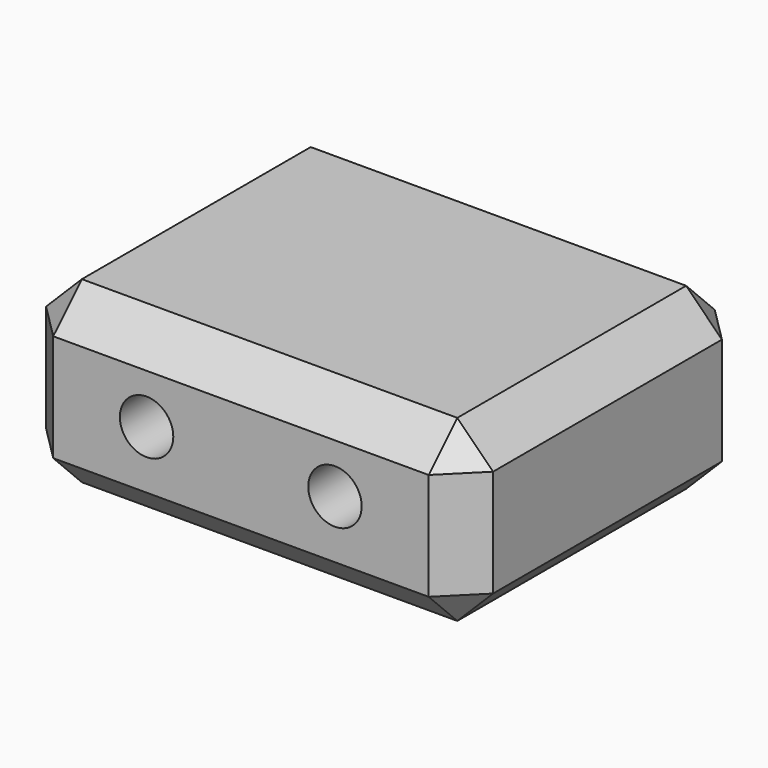
from build123d import *

# Parameters (mm, degrees)
F1_DEPTH = 5
F3_SIZE  = 1
F4_R     = 0.7470588235
F5_DEPTH = 7.5


# Not quite as in the source:
# - a feature names something its author has since deleted; it is built from what else it names


with BuildPart() as f1:
    # F0 (on Top) → F1 (new body)
    with BuildSketch(Plane.XY):
        Polygon((9.4699421152, -1.9223576039), (-3.0300578848, -1.9223576039), (-3.0300578848, -6.9223576039), (-3.0300578848, -11.9223576039), (9.4699421152, -11.9223576039), align=None)
    extrude(amount=F1_DEPTH)

    # F3
    f3_edges = [f1.edges().sort_by_distance(p)[0] for p in [
        (3.219942, -11.922358, 5),
        (9.469942, -6.922358, 5),
        (-3.030058, -1.922358, 2.5),
        (-3.030058, -11.922358, 2.5),
        (9.469942, -11.922358, 2.5),
        (9.469942, -6.922358, 0),
        (3.219942, -11.922358, 0),
        (9.469942, -1.922358, 2.5),
        (-3.030058, -6.922358, 5),
        (3.219942, -1.922358, 5),
        (3.219942, -1.922358, 0),
        (-3.030058, -6.922358, 0),
    ]]
    chamfer(f3_edges, length=F3_SIZE)

    # F4 (on face) → F5 (cut)
    with BuildSketch(Plane.XZ.offset(11.9223576039)):
        with Locations((0.5804465618, 2.6189445052)):
            Circle(F4_R)
        with Locations((5.8481891174, 2.6189445052)):
            Circle(F4_R)
    extrude(amount=-F5_DEPTH, mode=Mode.SUBTRACT)


solid = f1.part
